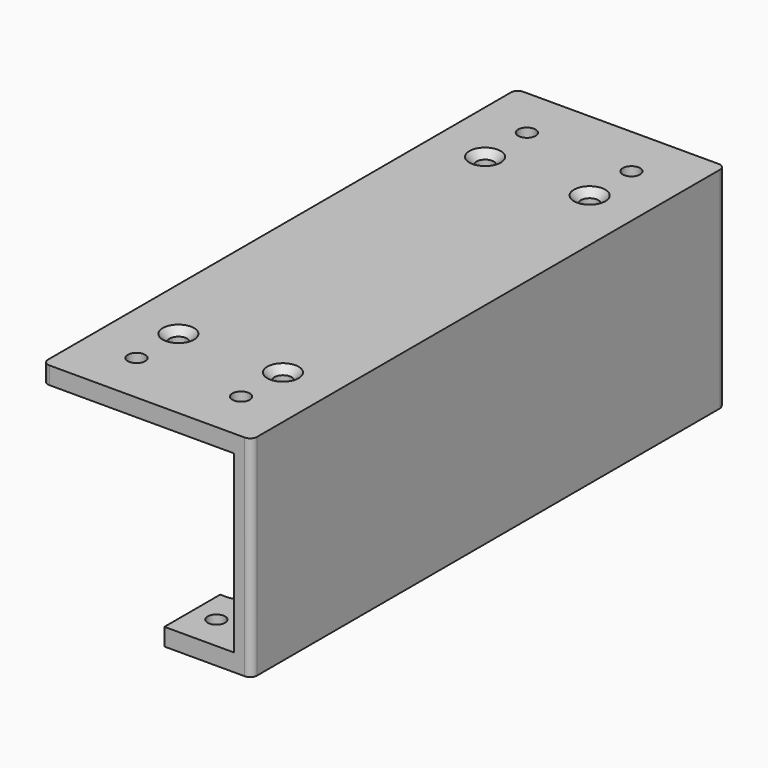
from build123d import *

# Parameters (mm, degrees)
F0_R     = 2.5
F1_DEPTH = 5
F2_W     = 170
F2_H     = 50.3
F3_DEPTH = 5
F4_W     = 55
F4_H     = 50.3
F5_DEPTH = 5
F7_R     = 2.5
F8_DEPTH = 5
F9_SIZE  = 2
F10_SIZE = 2
F11_SIZE = 2
F12_R    = 2


# Not quite as in the source:
# - a feature names something its author has since deleted; it is built from what else it names


with BuildPart() as f1:
    # F0 (on Top) → F1 (new body)
    with BuildSketch(Plane.XY):
        with BuildLine():
            Line((-60, 0), (0, 0))
            Line((0, 0), (0, 150))
            Line((0, 150), (0, 170))
            Line((0, 170), (-15, 170))
            add(Edge.make_bspline(
                [(-15, 170), (-14.4841735922, 160.0600889734), (-13.9683471845, 150.1201779469), (-13.6234299021, 140.3529161241)],
                knots=[0, 0, 0, 0, 0.0906883322, 0.0906883322, 0.0906883322, 0.0906883322], degree=3))
            add(Edge.make_bspline(
                [(-13.6234299021, 140.3529161241), (-12.0632834056, 96.1731661082), (-14.5980537911, 42.9711861088), (-50.2193379026, 23.1925838291), (-60, 19.9139873857)],
                knots=[0.0906883322, 0.0906883322, 0.0906883322, 0.0906883322, 0.5008941728, 0.6275927921, 0.6275927921, 0.6275927921, 0.6275927921], degree=3))
            Line((-60, 19.9139873857), (-60, 0))
        make_face()
        with Locations((-21.5087961406, 26.8674660474)):
            Circle(F0_R, mode=Mode.SUBTRACT)
        with BuildLine():
            ThreePointArc((-23.6172004723, 150), (-16.6720280929, 147.1947606368), (-13.6234299021, 140.3529161241))
            add(Edge.make_bspline(
                [(-15, 170), (-14.4841735922, 160.0600889734), (-13.9683471845, 150.1201779469), (-13.6234299021, 140.3529161241)],
                knots=[0, 0, 0, 0, 0.0906883322, 0.0906883322, 0.0906883322, 0.0906883322], degree=3))
            Line((-15, 170), (-25, 170))
            Line((-25, 170), (-25, 150))
            Line((-25, 150), (-23.6172004723, 150))
        make_face()
        with Locations((-18.0946737528, 160.0040644407)):
            Circle(F0_R, mode=Mode.SUBTRACT)
    extrude(amount=F1_DEPTH)

    # F2 (on face) → F3 (join)
    with BuildSketch(Plane.YZ):
        with Locations((85, 30.15)):
            Rectangle(F2_W, F2_H)
    extrude(amount=-F3_DEPTH)

    # F4 (on face) → F5 (join)
    with BuildSketch(Plane.XZ):
        with Locations((-32.5, 30.15)):
            Rectangle(F4_W, F4_H)
    extrude(amount=-F5_DEPTH)

    # F7 (on face) → F8 (join)
    with BuildSketch(Plane.XY.offset(55.3)):
        Polygon((-15, 0), (0, 0), (0, 15), (0, 155), (0, 170), (-15, 170), (-45, 170), (-60, 170), (-60, 155), (-60, 15), (-60, 0), (-45, 0), align=None)
        with Locations((-45, 15)):
            Circle(F7_R, mode=Mode.SUBTRACT)
        with Locations((-45, 30)):
            Circle(F7_R, mode=Mode.SUBTRACT)
        with Locations((-15, 15)):
            Circle(F7_R, mode=Mode.SUBTRACT)
        with Locations((-15, 30)):
            Circle(F7_R, mode=Mode.SUBTRACT)
        with Locations((-45, 140)):
            Circle(F7_R, mode=Mode.SUBTRACT)
        with Locations((-45, 155)):
            Circle(F7_R, mode=Mode.SUBTRACT)
        with Locations((-15, 140)):
            Circle(F7_R, mode=Mode.SUBTRACT)
        with Locations((-15, 155)):
            Circle(F7_R, mode=Mode.SUBTRACT)
    extrude(amount=F8_DEPTH)

    # F9
    f9_edges = [f1.edges().sort_by_distance(p)[0] for p in [
        (-17.5, 140, 60.3),
        (-47.5, 140, 60.3),
        (-17.5, 30, 60.3),
        (-47.5, 30, 60.3),
    ]]
    chamfer(f9_edges, length=F9_SIZE)

    # F10
    f10_edges = [f1.edges().sort_by_distance(p)[0] for p in [
        (-47.5, 155, 55.3),
        (-17.5, 155, 55.3),
        (-47.5, 15, 55.3),
        (-17.5, 15, 55.3),
    ]]
    chamfer(f10_edges, length=F10_SIZE)

    # F11
    f11_edges = [f1.edges().sort_by_distance(p)[0] for p in [
        (-24.008796, 26.867466, 0),
        (-20.594674, 160.004064, 0),
    ]]
    chamfer(f11_edges, length=F11_SIZE)

    # F12
    f12_edges = [f1.edges().sort_by_distance(p)[0] for p in [
        (0, 0, 30.15),
        (-60, 0, 30.15),
        (-30, 0, 0),
        (0, 170, 30.15),
        (-60, 170, 57.8),
    ]]
    fillet(f12_edges, radius=F12_R)


with BuildPart() as f13_1:
    # F13: instance of F1
    add(f1.part.mirror(Plane(origin=(-30, 0, 31.15), x_dir=(1, 0, 0), z_dir=(0, -1, 0))))


solid = f13_1.part
